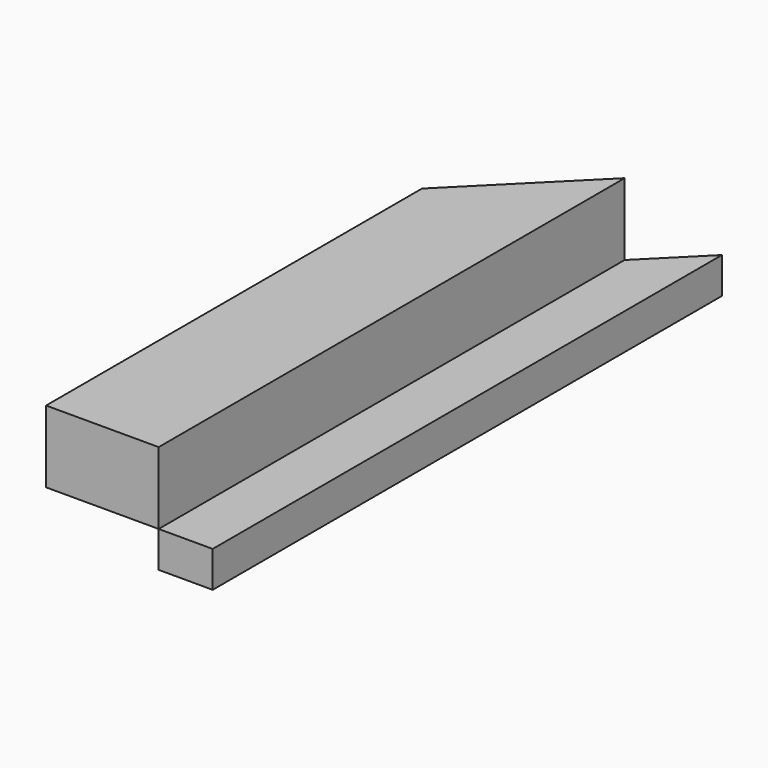
from build123d import *

# Parameters (mm, degrees)
F0_W        = 457.2
F0_H        = 304.8
F2_DEPTH    = 5410.2
F1_W        = 952.5
F1_H        = 609.6
F3_DEPTH    = 4927.6
F4_T1_DEPTH = 2786.9884199847
F5_SIZE     = 952.49999


# Not quite as in the source:
# - a fillet or chamfer that OpenCascade refuses, or shapes differently, is made with other operations: its cross-section is extruded or revolved along the edge and cut away or added
# - a fillet or chamfer is up to 0.001 mm smaller than in the source, because OpenCascade refuses the exact size


with BuildPart() as f2:
    # F0 (on Front) → F2 (new body)
    with BuildSketch(Plane.XZ):
        with Locations((228.6, 68.3558752648)):
            Rectangle(F0_W, F0_H)
    extrude(amount=-F2_DEPTH)

    # F4: chamfer of 482.6 on 1 edges, made by hand

    # F4_s2 → F4_t1 (cut)
    with BuildSketch(Plane.XY.offset(-1325.1383347275)):
        Polygon((0, 4927.6), (482.6, 5410.2), (0, 5410.2), align=None)
    extrude(amount=F4_T1_DEPTH, mode=Mode.SUBTRACT)


with BuildPart() as f3:
    # F1 (on face) → F3 (new body)
    with BuildSketch(Plane.XZ):
        with Locations((-476.25, 525.5558752648)):
            Rectangle(F1_W, F1_H)
    extrude(amount=-F3_DEPTH)

    # F5 (size 952.5 in the source; OpenCascade refuses exactly that, so slightly less here)
    f5_edges = [f3.edges().sort_by_distance(p)[0] for p in [
        (-952.5, 4927.6, 525.555875),
    ]]
    chamfer(f5_edges, length=F5_SIZE)


solid = Compound([f2.part, f3.part])
